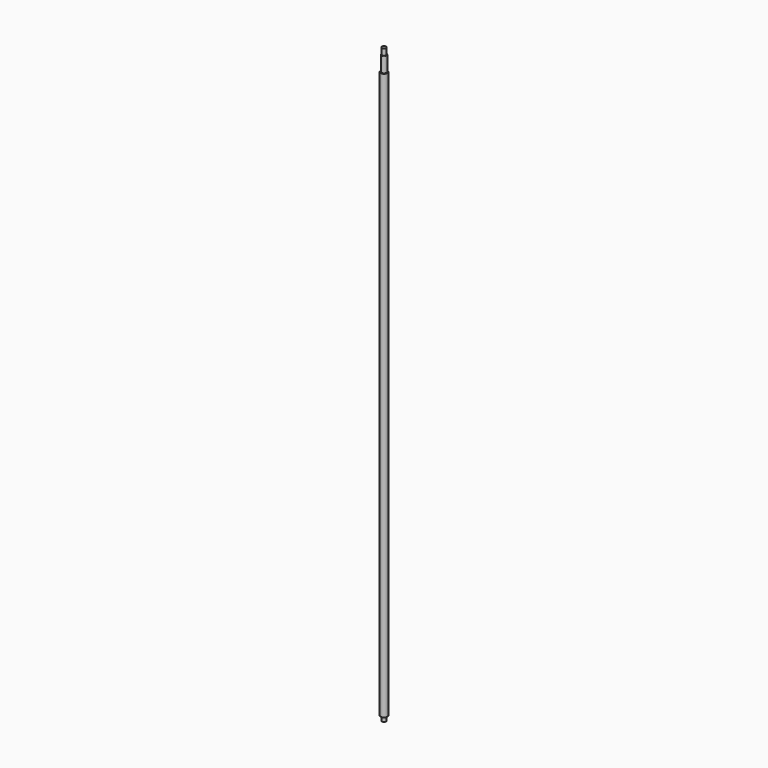
from build123d import *

# Parameters (mm, degrees)
F0_W   = 5
F0_H   = 15
F0_W_2 = 6
F0_H_2 = 22
F0_H_3 = 11
F3_R   = 0.2


# Not quite as in the source:
# - the program builds the solid bodies; features that only make, move or delete a surface that nothing else refers to are left out


with BuildPart() as f1:
    # F0 (on Front) → F1 (revolve)
    with BuildSketch(Plane.XZ):
        with Locations((2.5, 712.5)):
            Rectangle(F0_W, F0_H)
    revolve(axis=Axis((0, 0, -310.3163262457), (0, 0, -1)))



with BuildPart() as f1b:
    # F0 (on Front) → F1, piece 2 (revolve)
    with BuildSketch(Plane.XZ):
        with Locations((3, 680)):
            Rectangle(F0_W_2, F0_H_2)
        Polygon((0, 669), (0, 59.3673475087), (0, -669), (5, -669), (8.025, -669), (8.025, 669), (6, 669), align=None)
        with Locations((2.5, -674.5)):
            Rectangle(F0_W, F0_H_3)
    revolve(axis=Axis((0, 0, -310.3163262457), (0, 0, -1)))


with BuildPart() as f1_1:
    add(f1.part)

    add(f1b.part)  # F2 merges F1b
    # F0 (on Front) → F2 (revolve)
    with BuildSketch(Plane.XZ):
        Polygon((0, 705), (0, 691), (6, 691), (6, 705), (5, 705), align=None)
    revolve(axis=Axis((0, 0, 389.6836737543), (0, 0, 1)))

    # F3
    f3_edges = [f1_1.edges().sort_by_distance(p)[0] for p in [
        (-5, 0, -680),
    ]]
    fillet(f3_edges, radius=F3_R)


solid = f1_1.part
